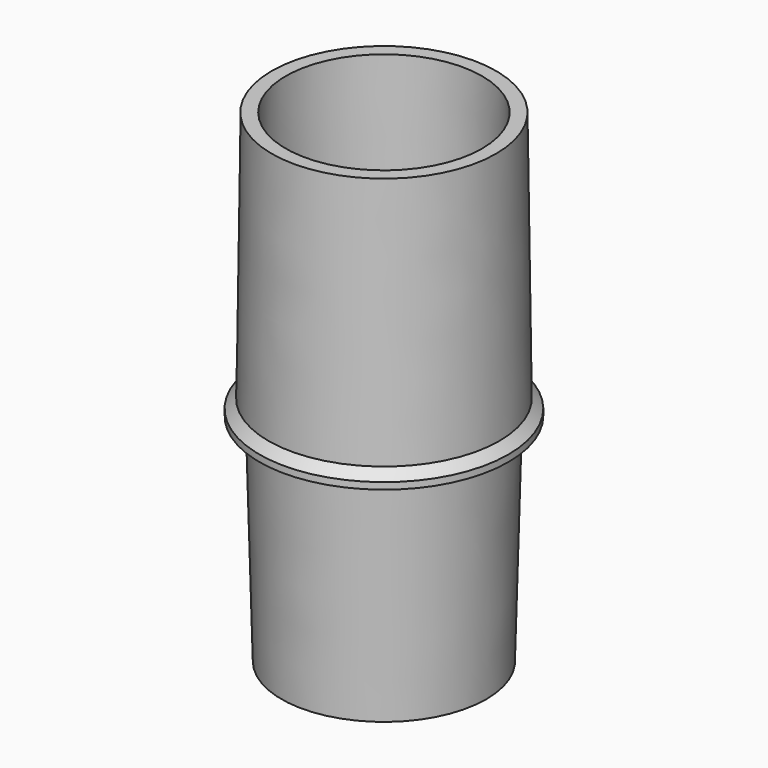
from build123d import *

# Parameters (mm, degrees)
F0_R      = 17.5
F0_R_2    = 15
F1_DEPTH  = 38.6
F1_TAPER  = -1.5
F2_R      = 22.25
F2_R_2    = 18.5107765726
F2_R_3    = 14
F3_DEPTH  = 2.8
F5_R      = 20.05
F5_R_2    = 17.55
F6_DEPTH  = 45
F6_TAPER  = -0.75
F7_SIZE   = 1.6109
F8_R      = 31.610490496
F9_DEPTH  = 38.6
F10_R     = 18.3
F10_R_2   = 15.8
F11_DEPTH = 38.6
F11_TAPER = -1.5


# Not quite as in the source:
# - a fillet or chamfer is up to 0.001 mm smaller than in the source, because OpenCascade refuses the exact size


with BuildPart() as f1:
    # F0 (on Top) → F1 (new body)
    with BuildSketch(Plane.XY):
        Circle(F0_R)
        Circle(F0_R_2, mode=Mode.SUBTRACT)
    extrude(amount=F1_DEPTH, taper=F1_TAPER)

    # F2 (on face) → F3 (join)
    with BuildSketch(Plane.XY.offset(38.6)):
        Circle(F2_R)
        Circle(F2_R_2, mode=Mode.SUBTRACT)
        Circle(F2_R_2)
        Circle(F2_R_3, mode=Mode.SUBTRACT)
    extrude(amount=F3_DEPTH)

    # F5 (on offset) → F6 (join, through all)
    with BuildSketch(Plane.XY.offset(86.4)):
        Circle(F5_R)
        Circle(F5_R_2, mode=Mode.SUBTRACT)
    extrude(amount=-F6_DEPTH, taper=F6_TAPER)

    # F7 (size 1.611 in the source; OpenCascade refuses exactly that, so slightly less here)
    f7_edges = [f1.edges().sort_by_distance(p)[0] for p in [
        (-22.25, 0, 41.4),
    ]]
    chamfer(f7_edges, length=F7_SIZE)

    # F8 (on Top) → F9 (cut, through all)
    with BuildSketch(Plane.XY):
        Circle(F8_R)
    extrude(amount=F9_DEPTH, mode=Mode.SUBTRACT)

    # F10 (on Top) → F11 (join, through all)
    with BuildSketch(Plane.XY):
        Circle(F10_R)
        Circle(F10_R_2, mode=Mode.SUBTRACT)
    extrude(amount=F11_DEPTH, taper=F11_TAPER)


solid = f1.part
